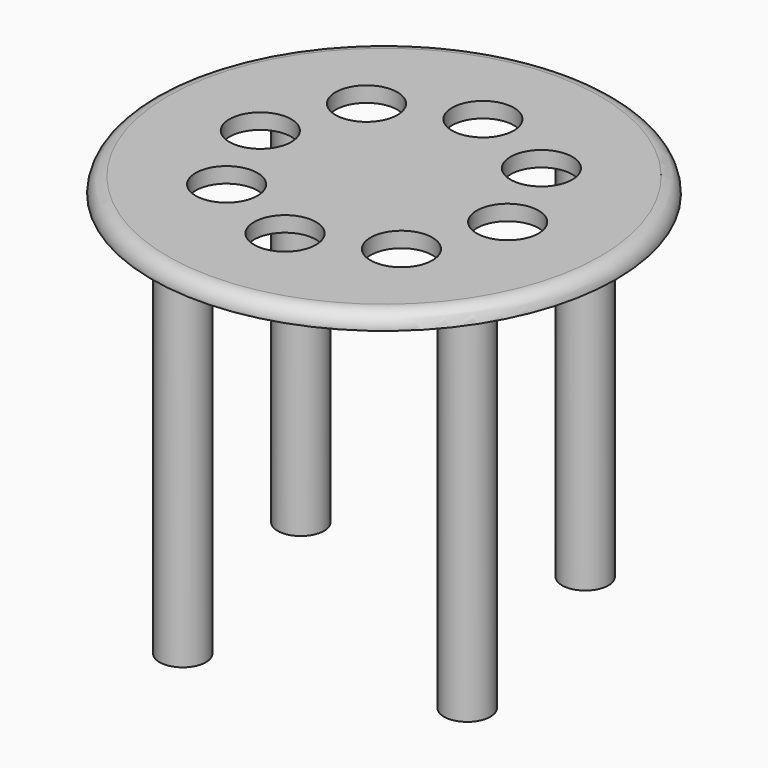
from build123d import *

# Parameters (mm, degrees)
F0_R     = 75
F0_R_2   = 10
F1_DEPTH = 5
F2_R     = 4.99999
F3_R     = 7.5
F4_DEPTH = 120


# Not quite as in the source:
# - a fillet or chamfer is up to 0.001 mm smaller than in the source, because OpenCascade refuses the exact size


with BuildPart() as f1:
    # F0 (on Top) → F1 (new body)
    with BuildSketch(Plane.XY):
        Circle(F0_R)
        with Locations((-28.2842712475, -28.2842712475)):
            Circle(F0_R_2, mode=Mode.SUBTRACT)
        with Locations((0, -40)):
            Circle(F0_R_2, mode=Mode.SUBTRACT)
        with Locations((28.2842712475, -28.2842712475)):
            Circle(F0_R_2, mode=Mode.SUBTRACT)
        with Locations((-40, 0)):
            Circle(F0_R_2, mode=Mode.SUBTRACT)
        with Locations((-28.2842712475, 28.2842712475)):
            Circle(F0_R_2, mode=Mode.SUBTRACT)
        with Locations((28.2842712475, 28.2842712475)):
            Circle(F0_R_2, mode=Mode.SUBTRACT)
        with Locations((40, 0)):
            Circle(F0_R_2, mode=Mode.SUBTRACT)
        with Locations((0, 40)):
            Circle(F0_R_2, mode=Mode.SUBTRACT)
    extrude(amount=F1_DEPTH)

    # F2 (radius 5 in the source; OpenCascade refuses exactly that, so slightly less here)
    f2_edges = [f1.edges().sort_by_distance(p)[0] for p in [
        (-75, 0, 5),
    ]]
    fillet(f2_edges, radius=F2_R)

    # F3 (on face) → F4 (join)
    with BuildSketch(Plane(origin=(0, 0, 0), x_dir=(1, 0, 0), z_dir=(0, 0, -1))):
        with Locations((-26.565498142, 48.1588445508)):
            Circle(F3_R)
        with Locations((-48.1588445508, -26.565498142)):
            Circle(F3_R)
        with Locations((26.565498142, -48.1588445508)):
            Circle(F3_R)
        with Locations((48.1588445508, 26.565498142)):
            Circle(F3_R)
    extrude(amount=F4_DEPTH)


solid = f1.part
